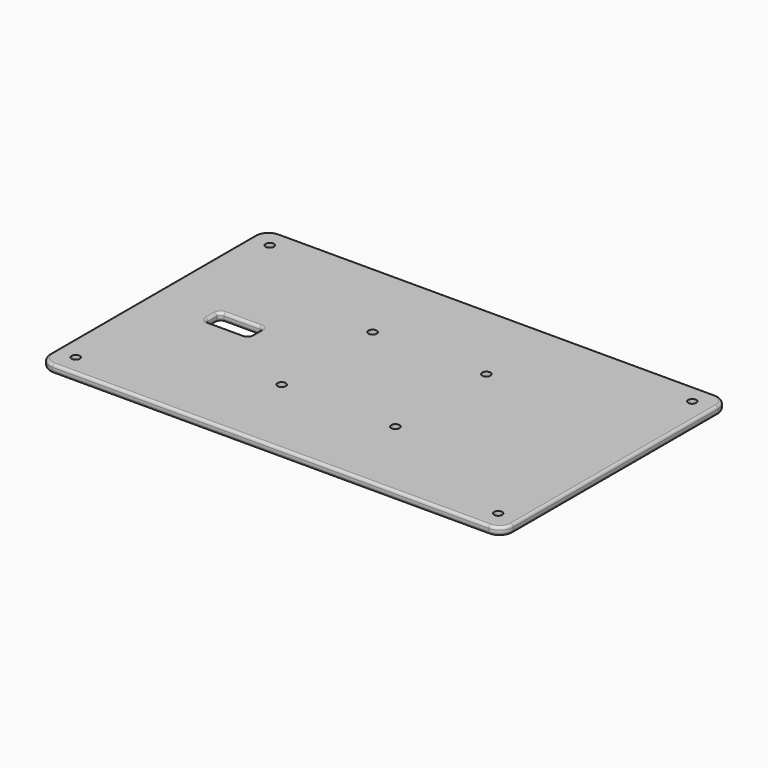
from build123d import *

# Parameters (mm, degrees)
F0_W     = 170
F0_H     = 104
F0_R     = 1.5
F0_R_2   = 2
F0_R_3   = 1.55
F0_W_2   = 16
F0_H_2   = 7
F1_DEPTH = 3
F2_R     = 5
F3_R     = 1.5
F4_R     = 1


with BuildPart() as f1:
    # F0 (on Top) → F1 (new body)
    with BuildSketch(Plane.XY):
        Rectangle(F0_W, F0_H)
        with Locations((-77.5, -44.5)):
            Circle(F0_R, mode=Mode.SUBTRACT)
        with Locations((-45, -40)):
            Circle(F0_R_2, mode=Mode.SUBTRACT)
        with Locations((-45, -30)):
            Circle(F0_R_2, mode=Mode.SUBTRACT)
        with Locations((-20.859650045, -20.859650045)):
            Circle(F0_R_3, mode=Mode.SUBTRACT)
        with Locations((77.5, -44.5)):
            Circle(F0_R, mode=Mode.SUBTRACT)
        with Locations((20.859650045, -20.859650045)):
            Circle(F0_R_3, mode=Mode.SUBTRACT)
        with Locations((-55, 0)):
            Rectangle(F0_W_2, F0_H_2, mode=Mode.SUBTRACT)
        with Locations((-20.859650045, 20.859650045)):
            Circle(F0_R_3, mode=Mode.SUBTRACT)
        with Locations((-45, 30)):
            Circle(F0_R_2, mode=Mode.SUBTRACT)
        with Locations((-77.5, 44.5)):
            Circle(F0_R, mode=Mode.SUBTRACT)
        with Locations((-45, 40)):
            Circle(F0_R_2, mode=Mode.SUBTRACT)
        with Locations((-10, 46)):
            Circle(F0_R_2, mode=Mode.SUBTRACT)
        with Locations((20.859650045, 20.859650045)):
            Circle(F0_R_3, mode=Mode.SUBTRACT)
        with Locations((0, 46)):
            Circle(F0_R_2, mode=Mode.SUBTRACT)
        with Locations((10, 46)):
            Circle(F0_R_2, mode=Mode.SUBTRACT)
        with Locations((77.5, 44.5)):
            Circle(F0_R, mode=Mode.SUBTRACT)
        with Locations((-45, 40)):
            Circle(F0_R_2)
        with Locations((-45, 30)):
            Circle(F0_R_2)
        with Locations((-45, -30)):
            Circle(F0_R_2)
        with Locations((-45, -40)):
            Circle(F0_R_2)
        with Locations((10, 46)):
            Circle(F0_R_2)
        with Locations((-10, 46)):
            Circle(F0_R_2)
        with Locations((0, 46)):
            Circle(F0_R_2)
    extrude(amount=F1_DEPTH)

    # F2
    f2_edges = [f1.edges().sort_by_distance(p)[0] for p in [
        (-85, -52, 1.5),
        (-85, 52, 1.5),
        (85, 52, 1.5),
        (85, -52, 1.5),
    ]]
    fillet(f2_edges, radius=F2_R)

    # F3
    f3_edges = [f1.edges().sort_by_distance(p)[0] for p in [
        (-47, 3.5, 1.5),
        (-47, -3.5, 1.5),
        (-63, -3.5, 1.5),
        (-63, 3.5, 1.5),
    ]]
    fillet(f3_edges, radius=F3_R)

    # F4
    f4_edges = [f1.edges().sort_by_distance(p)[0] for p in [
        (0, 52, 3),
        (0, 52, 0),
        (-55, -3.5, 3),
        (-55, 3.5, 0),
        (-55, -3.5, 0),
        (-47.43934, -3.06066, 0),
        (-62.56066, -3.06066, 0),
        (-47, 0, 0),
        (-63, 0, 0),
        (-47.43934, 3.06066, 0),
        (-62.56066, 3.06066, 0),
        (83.535534, 50.535534, 0),
        (-83.535534, 50.535534, 0),
        (85, 0, 0),
        (-85, 0, 0),
        (83.535534, -50.535534, 0),
        (-83.535534, -50.535534, 0),
        (0, -52, 0),
        (-47.43934, -3.06066, 3),
        (-62.56066, -3.06066, 3),
        (-47, 0, 3),
        (-63, 0, 3),
        (-47.43934, 3.06066, 3),
        (-62.56066, 3.06066, 3),
        (-55, 3.5, 3),
        (83.535534, 50.535534, 3),
        (-83.535534, 50.535534, 3),
        (85, 0, 3),
        (-85, 0, 3),
        (83.535534, -50.535534, 3),
        (-83.535534, -50.535534, 3),
        (0, -52, 3),
    ]]
    fillet(f4_edges, radius=F4_R)


solid = f1.part
